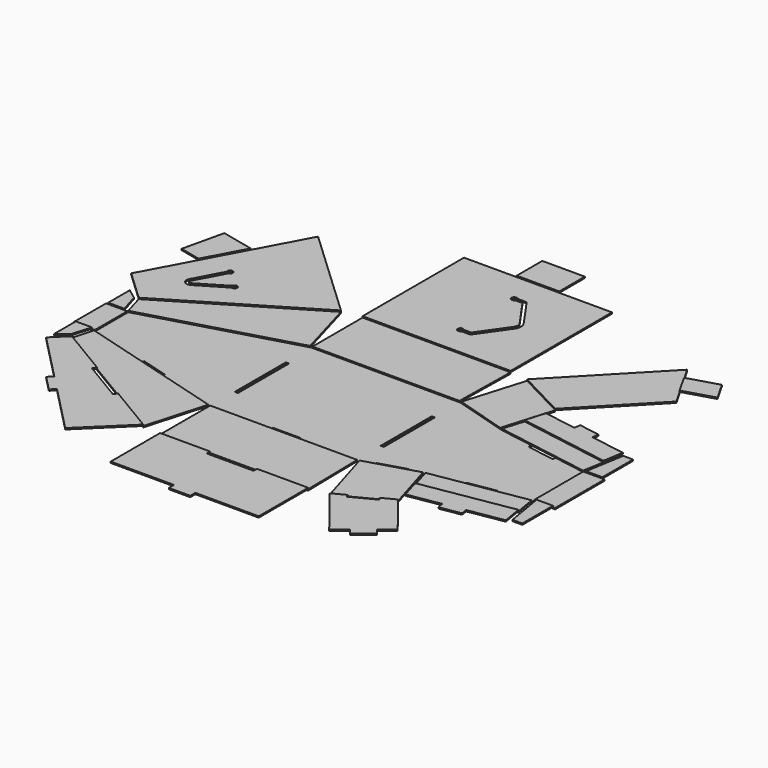
from build123d import *

# Parameters (mm, degrees)
F1_DEPTH  = 0.6
F3_DEPTH  = 0.6
F5_DEPTH  = 0.6
F7_DEPTH  = 0.6
F9_DEPTH  = 0.6
F10_W     = 10
F10_H     = 19
F11_DEPTH = 0.6
F12_W     = 10
F12_H     = 29
F13_DEPTH = 0.6
F15_DEPTH = 0.6
F17_DEPTH = 0.6
F19_DEPTH = 25
F21_DEPTH = 0.6
F22_W     = 20
F22_H     = 15
F23_DEPTH = 0.6
F25_DEPTH = 0.6
F27_DEPTH = 0.6
F28_W     = 12.9999998421
F28_H     = 1.5
F29_DEPTH = 25
F31_DEPTH = 0.6
F33_DEPTH = 25
F35_DEPTH = 25
F37_DEPTH = 0.6
F39_DEPTH = 0.6
F41_DEPTH = 0.6
F43_DEPTH = 0.6
F45_DEPTH = 0.6
F47_DEPTH = 25
F49_DEPTH = 25
F51_DEPTH = 25
F53_DEPTH = 25
F54_W     = 1.5
F54_H     = 30
F55_DEPTH = 25


with BuildPart() as f1:
    # F0 (on Top) → F1 (new body)
    with BuildSketch(Plane.XY):
        Polygon((35, 30), (-35, 30), (-105, 10), (-105, 0), (-105, -10), (-35, -30), (35, -30), (60, -22.5), (105, -15), (105, 0), (105, 15), (60, 22.5), align=None)
    extrude(amount=-F1_DEPTH)

    # F18 (on face) → F19 (cut)
    with BuildSketch(Plane.XY):
        Polygon((89.2912438804, 16.0974353874), (89.5378423613, 17.5770262731), (76.714718837, 19.7142135272), (76.468120356, 18.2346226414), align=None)
        Polygon((89.5378423613, -17.5770262731), (89.2912438804, -16.0974353874), (76.468120356, -18.2346226414), (76.714718837, -19.7142135272), align=None)
    extrude(amount=-F19_DEPTH, mode=Mode.SUBTRACT)

    # F28 (on face) → F29 (cut)
    with BuildSketch(Plane.XY):
        with Locations((0.251774159, -29.25)):
            Rectangle(F28_W, F28_H)
    extrude(amount=-F29_DEPTH, mode=Mode.SUBTRACT)

    # F32 (on face) → F33 (cut)
    with BuildSketch(Plane.XY):
        Polygon((-76.0782049547, -16.7033464652), (-76.4902866466, -18.1456323867), (-63.9904753272, -21.7170070494), (-63.5783936354, -20.2747211279), align=None)
    extrude(amount=-F33_DEPTH, mode=Mode.SUBTRACT)

    # F48 (on face) → F49 (cut)
    with BuildSketch(Plane.XY):
        Polygon((41.2741291461, -28.1177612562), (53.7258708539, -24.3822387438), (53.2948490256, -22.945499316), (40.8431073177, -26.6810218283), align=None)
    extrude(amount=-F49_DEPTH, mode=Mode.SUBTRACT)

    # F54 (on face) → F55 (cut)
    with BuildSketch(Plane.XY):
        with Locations((-34.25, 0)):
            Rectangle(F54_W, F54_H)
        with Locations((34.25, 0)):
            Rectangle(F54_W, F54_H)
    extrude(amount=-F55_DEPTH, mode=Mode.SUBTRACT)


with BuildPart() as f3:
    # F2 (on face) → F3 (new body)
    with BuildSketch(Plane.XY):
        Polygon((-35.4807619738, -29.8626394361), (-105, -10), (-107.747211279, -19.6152394764), (-43.5182780127, -57.9939455722), align=None)
    extrude(amount=F3_DEPTH)


with BuildPart() as f3b:
    # F2 (on face) → F3, piece 2 (new body)
    with BuildSketch(Plane.XY):
        Polygon((-107.747211279, 19.6152394764), (-105, 10), (-35.4807619738, 29.8626394361), (-43.5182780127, 57.9939455722), align=None)
    extrude(amount=F3_DEPTH)


with BuildPart() as f5:
    # F4 (on face) → F5 (new body)
    with BuildSketch(Plane.XY):
        Polygon((-34.5, 30), (34.5, 30), (35, 59.3957479918), (-34.5, 59.4), align=None)
    extrude(amount=F5_DEPTH)


with BuildPart() as f5b:
    # F4 (on face) → F5, piece 2 (new body)
    with BuildSketch(Plane.XY):
        Polygon((34.5, -30), (-34.5, -30), (-34.5, -59.4), (35, -59.3957479918), align=None)
    extrude(amount=F5_DEPTH)


with BuildPart() as f7:
    # F6 (on face) → F7 (new body)
    with BuildSketch(Plane.XY):
        Polygon((66.5611100538, -46.1104179307), (59.5210868574, -22.6436739428), (35.4789131426, -29.8563260572), (43.8982061897, -57.9206362142), align=None)
    extrude(amount=F7_DEPTH)


with BuildPart() as f7b:
    # F6 (on face) → F7, piece 2 (new body)
    with BuildSketch(Plane.XY):
        Polygon((35.4789131426, 29.8563260572), (59.5210868574, 22.6436739428), (66.5611100538, 46.1104179307), (43.8982061897, 57.9206362142), align=None)
    extrude(amount=F7_DEPTH)


with BuildPart() as f9:
    # F8 (on face) → F9 (new body)
    with BuildSketch(Plane.XY):
        Polygon((106.1507929111, -24.946138732), (104.5068030381, -15.0821994937), (60.4931969619, -22.4178005063), (63.3897505478, -32.0729791259), align=None)
    extrude(amount=F9_DEPTH)


with BuildPart() as f9b:
    # F8 (on face) → F9, piece 2 (new body)
    with BuildSketch(Plane.XY):
        Polygon((60.4931969619, 22.4178005063), (104.5068030381, 15.0821994937), (106.1507929111, 24.946138732), (63.3897505478, 32.0729791259), align=None)
    extrude(amount=F9_DEPTH)


with BuildPart() as f11:
    # F10 (on face) → F11 (new body)
    with BuildSketch(Plane.XY):
        with Locations((-110, 0)):
            Rectangle(F10_W, F10_H)
    extrude(amount=F11_DEPTH)


with BuildPart() as f13:
    # F12 (on face) → F13 (new body)
    with BuildSketch(Plane.XY):
        with Locations((110, 0)):
            Rectangle(F12_W, F12_H)
    extrude(amount=F13_DEPTH)


with BuildPart() as f15:
    # F14 (on face) → F15 (new body)
    with BuildSketch(Plane.XY.offset(0.6)):
        Polygon((63.3897505478, 32.0729791259), (106.1507929111, 24.946138732), (107.7125832905, 34.3168810084), (91.264031728, 37.0583062688), (91.7572286899, 40.0174880403), (86.8252590708, 40.8394829768), (81.8932869371, 41.6614783324), (81.4000899752, 38.7022965609), (66.1414764543, 41.2453988144), align=None)
    extrude(amount=F15_DEPTH)


with BuildPart() as f15b:
    # F14 (on face) → F15, piece 2 (new body)
    with BuildSketch(Plane.XY.offset(0.6)):
        Polygon((91.7572286899, -40.0174880403), (91.264031728, -37.0583062688), (107.7125832905, -34.3168810084), (106.1507929111, -24.946138732), (63.3897505478, -32.0729791259), (66.1414764543, -41.2453988144), (81.4000899752, -38.7022965609), (81.8932869371, -41.6614783324), (86.8252590708, -40.8394829768), align=None)
    extrude(amount=F15_DEPTH)


with BuildPart() as f17:
    # F16 (on face) → F17 (new body)
    with BuildSketch(Plane.XY.offset(0.6)):
        Polygon((106.3502579927, 14.5), (115, 14.5), (115, 32.5), (109.3824233932, 32.5), align=None)
    extrude(amount=F17_DEPTH)


with BuildPart() as f17b:
    # F16 (on face) → F17, piece 2 (new body)
    with BuildSketch(Plane.XY.offset(0.6)):
        Polygon((115, -32.5), (115, -14.5), (106.3502579927, -14.5), (109.3824233932, -32.5), align=None)
    extrude(amount=F17_DEPTH)


with BuildPart() as f21:
    # F20 (on face) → F21 (new body)
    with BuildSketch(Plane.XY.offset(0.6)):
        Polygon((-34.4963597916, 118.8999998886), (-34.5, 59.4), (35, 59.3957479918), (35.0036402084, 118.8957478805), align=None)
    extrude(amount=F21_DEPTH)

    # F50 (on face) → F51 (cut)
    with BuildSketch(Plane.XY.offset(1.2)):
        with BuildLine():
            Line((1.2527378019, 104.1478127322), (4.7467792496, 104.1475989668))
            Line((4.7467792496, 104.1475989668), (14.0469048874, 90.8681254198))
            ThreePointArc((14.0469048874, 90.8681254198), (14.5895998787, 89.1469967553), (14.0466942942, 87.4259345077))
            Line((14.0466942942, 87.4259345077), (4.7449438504, 74.147599023))
            Line((4.7449438504, 74.147599023), (1.2509024027, 74.1478127883))
            ThreePointArc((1.2509024027, 74.1478127883), (-0.999143478, 73.3979504447), (1.2508106328, 72.6478127912))
            Line((1.2508106328, 72.6478127912), (5.5255606239, 72.6475512621))
            Line((5.5255606239, 72.6475512621), (15.2752414992, 86.565311614))
            ThreePointArc((15.2752414992, 86.565311614), (16.0895998759, 89.1469049853), (15.2755573889, 91.7285979821))
            Line((15.2755573889, 91.7285979821), (5.527579563, 105.6475512003))
            Line((5.527579563, 105.6475512003), (1.2528295719, 105.6478127294))
            ThreePointArc((1.2528295719, 105.6478127294), (-0.9972163089, 104.8979503857), (1.2527378019, 104.1478127322))
        make_face()
    extrude(amount=-F51_DEPTH, mode=Mode.SUBTRACT)


with BuildPart() as f23:
    # F22 (on face) → F23 (new body)
    with BuildSketch(Plane.XY.offset(1.2)):
        with Locations((0.2536402084, 126.3978738846)):
            Rectangle(F22_W, F22_H)
    extrude(amount=F23_DEPTH)


with BuildPart() as f25:
    # F24 (on face) → F25 (new body)
    with BuildSketch(Plane.XY.offset(0.6)):
        Polygon((-10.9963660181, -59.3985620483), (-34.5, -59.4), (-34.4982257808, -88.3999999457), (-4.7482257621, -88.3981798415), (-4.7482257621, -91.3981798415), (5.25177408, -91.3981798415), (5.25177408, -88.3975680418), (35.0017742192, -88.3957479376), (35, -59.3957479918), (11.0036339407, -59.3972160889), (11.0037564298, -61.3993270166), (0.0037564504, -61.3999999963), (-10.996243529, -61.400672976), align=None)
    extrude(amount=F25_DEPTH)


with BuildPart() as f27:
    # F26 (on face) → F27 (new body)
    with BuildSketch(Plane.XY.offset(0.6)):
        Polygon((-121.9631661268, 32.9627721234), (-107.747211279, 19.6152394764), (-43.5182780127, 57.9939455722), (-86.6946844673, 98.5327979322), align=None)
    extrude(amount=F27_DEPTH)

    # F52 (on face) → F53 (cut)
    with BuildSketch(Plane.XY.offset(1.2)):
        with BuildLine():
            Line((-101.2073088148, 41.9967839558), (-94.1454949769, 55.1258809233))
            ThreePointArc((-94.1454949769, 55.1258809233), (-93.740186363, 57.4627003274), (-95.4665248966, 55.8364299725))
            Line((-95.4665248966, 55.8364299725), (-102.5283387344, 42.707333005))
            ThreePointArc((-102.5283387344, 42.707333005), (-102.0540667173, 39.7158946591), (-99.0442827829, 39.3770171128))
            Line((-99.0442827829, 39.3770171128), (-86.1525430441, 47.0802166732))
            ThreePointArc((-86.1525430441, 47.0802166732), (-84.6057841406, 48.8781423931), (-86.9219466954, 48.3678571593))
            Line((-86.9219466954, 48.3678571593), (-99.8136864341, 40.6646575989))
            ThreePointArc((-99.8136864341, 40.6646575989), (-101.0176000079, 40.8002086174), (-101.2073088148, 41.9967839558))
        make_face()
    extrude(amount=-F53_DEPTH, mode=Mode.SUBTRACT)


with BuildPart() as f31:
    # F30 (on face) → F31 (new body)
    with BuildSketch(Plane.XY.offset(0.6)):
        Polygon((-85.0754415438, -33.1622990816), (-107.747211279, -19.6152394764), (-114.5548071354, -26.2414479439), (-92.8284731165, -48.5583412531), (-94.9780442288, -50.6510294843), (-88.0024162111, -57.8162671218), (-85.8528450987, -55.7235788906), (-64.1265116603, -78.0404716036), (-43.5182780127, -57.9939455722), (-66.1900477479, -44.446885967), (-67.2159192829, -46.1637399484), (-86.1013130788, -34.8791530631), align=None)
    extrude(amount=F31_DEPTH)


with BuildPart() as f35_tool:
    # F34 (on face) → F35 (new body)
    with BuildSketch(Plane.XY.offset(1.2)):
        Polygon((114, 14.5), (115, 14.5), (115, -14.5), (114, -14.5), (114, -39.447799325), (116.3519918919, -36.2990759313), (116.3519918919, 33.8478907943), (114, 33.8478907943), align=None)
    extrude(amount=-F35_DEPTH)


with BuildPart() as f17_1:
    add(f17.part)

    # F35: cut by f35_tool
    add(f35_tool.part, mode=Mode.SUBTRACT)


with BuildPart() as f17b_1:
    add(f17b.part)

    # F35: cut by f35_tool
    add(f35_tool.part, mode=Mode.SUBTRACT)


with BuildPart() as f37:
    # F36 (on face) → F37 (new body)
    with BuildSketch(Plane.XY.offset(1.2)):
        Polygon((-109.2414129666, 56.6146460857), (-99.4164376275, 74.88092397), (-114.5188272623, 78.3436335989), (-118.988490831, 58.8494778701), align=None)
    extrude(amount=F37_DEPTH)


with BuildPart() as f39:
    # F38 (on face) → F39 (new body)
    with BuildSketch(Plane.XY.offset(0.6)):
        Polygon((-114, 22.1587866545), (-114, 9.5), (-106.3893288374, 9.5), (-109.1255843639, 18.5674559325), align=None)
    extrude(amount=F39_DEPTH)


with BuildPart() as f39b:
    # F38 (on face) → F39, piece 2 (new body)
    with BuildSketch(Plane.XY.offset(0.6)):
        Polygon((-114, -9.5), (-114, -22.1587866545), (-109.1255843639, -18.5674559325), (-106.3893288374, -9.5), align=None)
    extrude(amount=F39_DEPTH)


with BuildPart() as f41:
    # F40 (on face) → F41 (new body)
    with BuildSketch(Plane.XY.offset(0.6)):
        Polygon((81.4526222314, -64.9317586126), (66.5611100538, -46.1104179307), (43.8982061897, -57.9206362142), (61.7680208029, -80.5062450325), (67.6892049249, -75.8213952003), (69.5506409516, -78.1740651556), (77.3928748081, -71.9692778683), (75.5314387815, -69.6166079129), align=None)
    extrude(amount=F41_DEPTH)

    # F46 (on face) → F47 (cut)
    with BuildSketch(Plane.XY.offset(1.2)):
        Polygon((61.2437128477, -50.5729093986), (60.55050547, -49.2426975616), (49.9088107735, -54.7883565833), (50.6020181512, -56.1185684204), align=None)
    extrude(amount=-F47_DEPTH, mode=Mode.SUBTRACT)


with BuildPart() as f43:
    # F42 (on face) → F43 (new body)
    with BuildSketch(Plane.XY.offset(0.6)):
        Polygon((84.9611208524, 100.5642411205), (43.8982061897, 57.9206362142), (66.5611100538, 46.1104179307), (97.6218755705, 78.3668474528), align=None)
    extrude(amount=F43_DEPTH)


with BuildPart() as f45:
    # F44 (on face) → F45 (new body)
    with BuildSketch(Plane.XY.offset(1.2)):
        Polygon((103.1165153293, 98.2331381751), (88.7491006834, 93.922987784), (93.8338938857, 85.0081040395), (108.2013085316, 89.3182544305), align=None)
    extrude(amount=F45_DEPTH)


solid = Compound([f1.part, f3.part, f3b.part, f5.part, f5b.part, f7.part, f7b.part, f9.part, f9b.part, f11.part, f13.part, f15.part, f15b.part, f21.part, f23.part, f25.part, f27.part, f31.part, f17_1.part, f17b_1.part, f37.part, f39.part, f39b.part, f41.part, f43.part, f45.part])
